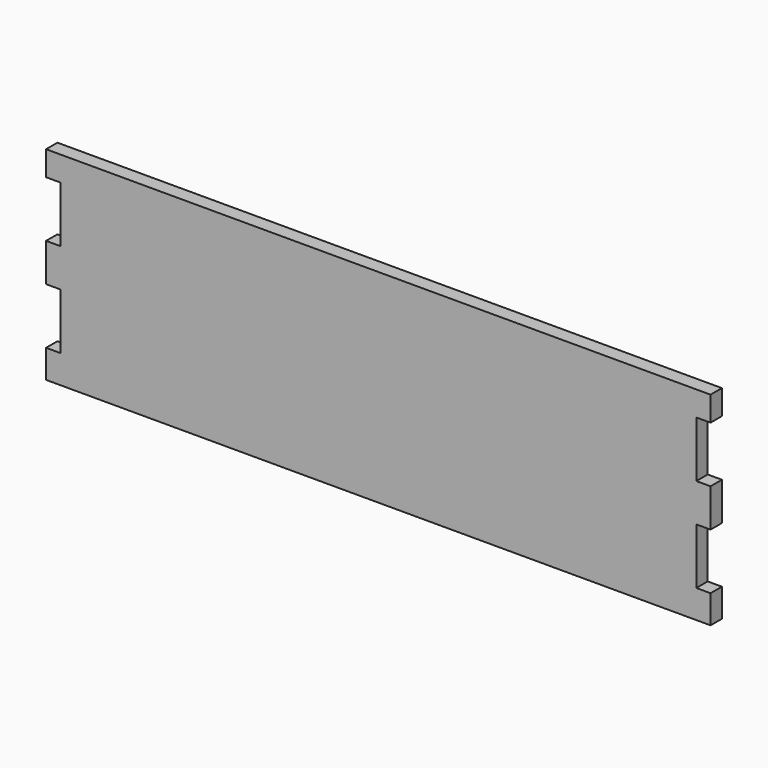
from build123d import *

# Parameters (mm, degrees)
F1_DEPTH = 3.81


# Not quite as in the source:
# - a feature names something its author has since deleted; it is built from what else it names


with BuildPart() as f1:
    # F0 (on Front) → F1 (new body)
    with BuildSketch(Plane.XZ):
        Polygon((89, 20.5917087717), (89, 27.203), (82.18, 27.203), (64, 27.203), (54, 27.203), (39, 27.203), (0, 27.203), (0, 0), (89, 0), (89, 5.5917087717), (85.19, 5.5917087717), (85.19, 20.5917087717), align=None)
        Polygon((-89, 0), (0, 0), (0, 27.203), (-39, 27.203), (-54, 27.203), (-64, 27.203), (-82.18, 27.203), (-89, 27.203), (-89, 20.5917087717), (-85.19, 20.5917087717), (-85.19, 5.5917087717), (-89, 5.5917087717), align=None)
        Polygon((0, -27.203), (0, 0), (-89, 0), (-89, -4.6252912283), (-85.19, -4.6252912283), (-85.19, -19.6252912283), (-89, -19.6252912283), (-89, -27.203), (-82.18, -27.203), (-64, -27.203), (-54, -27.203), (-39, -27.203), align=None)
        Polygon((89, -4.6252912283), (89, 0), (0, 0), (0, -27.203), (39, -27.203), (54, -27.203), (64, -27.203), (82.18, -27.203), (89, -27.203), (89, -19.6252912283), (85.19, -19.6252912283), (85.19, -4.6252912283), align=None)
    extrude(amount=F1_DEPTH)


solid = f1.part
